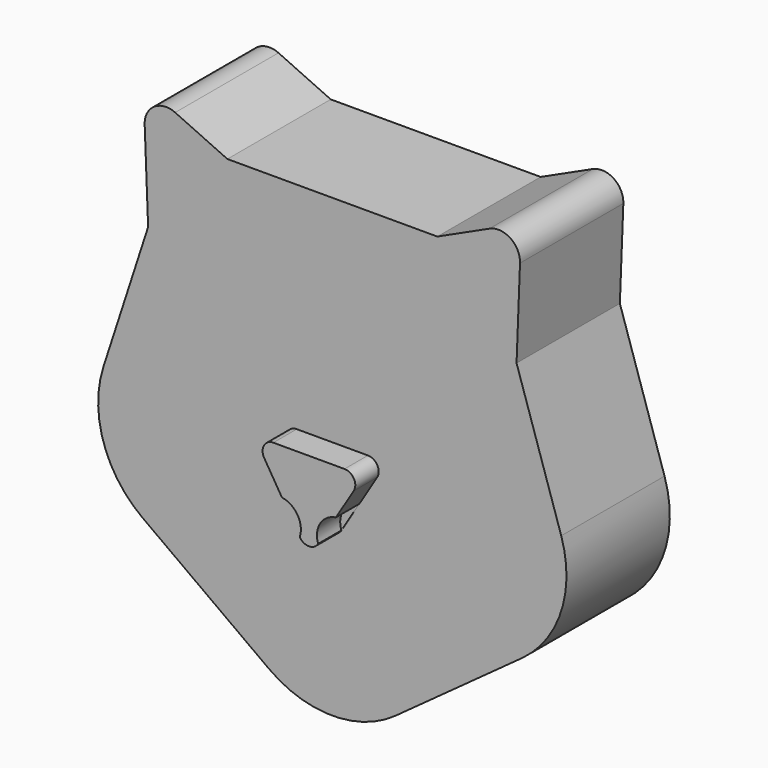
from build123d import *

# Parameters (mm, degrees)
F1_DEPTH  = 6
F3_DEPTH  = 6
F5_R      = 2
F6_R      = 10
F9_DEPTH  = 2.7195
F10_R     = 1
F18_DEPTH = 2.7


# Not quite as in the source:
# - the program builds the solid bodies; features that only make, move or delete a surface that nothing else refers to are left out


with BuildPart() as f1:
    # F0 (on Front) → F1 (new body, symmetric)
    with BuildSketch(Plane.XZ):
        Polygon((-23.5114100917, -7.639320225), (0, -24.72135955), (23.5114100917, -7.639320225), (14.5308505601, 20), (-14.5308505601, 20), align=None)
    extrude(amount=F1_DEPTH, both=True)

    # F2 (on Front) → F3 (join, symmetric)
    with BuildSketch(Plane.XZ):
        Polygon((-17.5627600402, 23.5819537193), (-17.116108973, 12.0433927434), (-9.7525370519, 20), align=None)
        Polygon((17.5627600402, 23.5819537193), (9.7525370519, 20), (17.116108973, 12.0433927434), align=None)
    extrude(amount=F3_DEPTH, both=True)

    # F5
    f5_edges = [f1.edges().sort_by_distance(p)[0] for p in [
        (-17.56276, 0, 23.581954),
        (17.56276, 0, 23.581954),
    ]]
    fillet(f5_edges, radius=F5_R)

    # F6
    f6_edges = [f1.edges().sort_by_distance(p)[0] for p in [
        (-23.51141, 0, -7.63932),
        (23.51141, 0, -7.63932),
        (0, 0, -24.72136),
    ]]
    fillet(f6_edges, radius=F6_R)

    # F8 (on face) → F9 (join)
    with BuildSketch(Plane.XZ.offset(6)):
        Polygon((5.0926953554, 0), (-5.0926953554, 0), (0, -8.3154477179), align=None)
    extrude(amount=F9_DEPTH)

    # F10
    f10_edges = [f1.edges().sort_by_distance(p)[0] for p in [
        (0, -7.35975, -8.315448),
        (-5.092695, -7.35975, 0),
        (5.092695, -7.35975, 0),
    ]]
    fillet(f10_edges, radius=F10_R)

    # F17 (on face) → F18 (cut)
    with BuildSketch(Plane.XZ.offset(8.7195)):
        with BuildLine():
            Line((0.8527780007, -6.9230159338), (2.5065876623, -4.2226447518))
            ThreePointArc((2.5065876623, -4.2226447518), (1.0499427142, -5.1871536265), (0.8527780007, -6.9230159338))
        make_face()
        with BuildLine():
            Line((-2.5065876623, -4.2226447518), (-0.8527780007, -6.9230159338))
            ThreePointArc((-0.8527780007, -6.9230159338), (-1.0499427142, -5.1871536265), (-2.5065876623, -4.2226447518))
        make_face()
    extrude(amount=-F18_DEPTH, mode=Mode.SUBTRACT)


solid = f1.part
